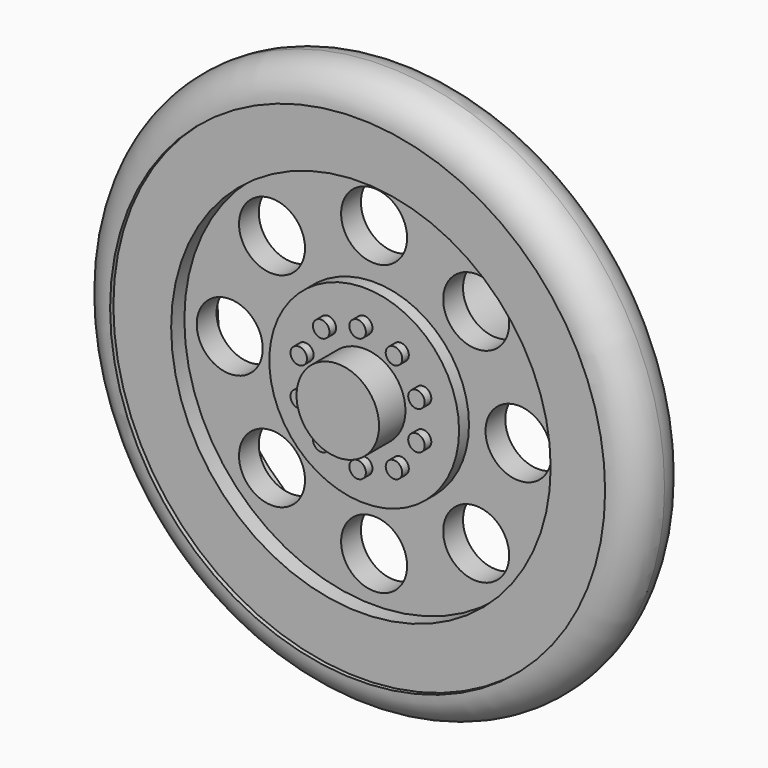
from build123d import *

# Parameters (mm, degrees)
F0_R      = 17
F1_DEPTH  = 4
F2_R      = 2
F3_R      = 1.99999
F4_R      = 15
F4_R_2    = 2
F4_R_3    = 5.75
F5_DEPTH  = 0.25
F6_DEPTH  = 0.25
F7_R      = 11.5
F7_R_2    = 2
F7_R_3    = 5.75
F8_DEPTH  = 1
F9_R      = 11.5
F10_DEPTH = 1
F11_DEPTH = 5
F12_DEPTH = 0.5
F13_R     = 0.5
F14_DEPTH = 0.5
F13_R_2   = 2.5
F15_DEPTH = 2
F16_R     = 3
F17_DEPTH = 8.5
F18_R     = 1.5
F19_DEPTH = 9


# Not quite as in the source:
# - a fillet or chamfer is up to 0.001 mm smaller than in the source, because OpenCascade refuses the exact size


with BuildPart() as f1:
    # F0 (on Front) → F1 (new body)
    with BuildSketch(Plane.XZ):
        Circle(F0_R)
    extrude(amount=F1_DEPTH)

    # F2
    f2_edges = [f1.edges().sort_by_distance(p)[0] for p in [
        (-17, -4, 0),
    ]]
    fillet(f2_edges, radius=F2_R)

    # F3 (radius 2 in the source; OpenCascade refuses exactly that, so slightly less here)
    f3_edges = [f1.edges().sort_by_distance(p)[0] for p in [
        (-17, 0, 0),
    ]]
    fillet(f3_edges, radius=F3_R)

    # F4 (on face) → F5 (cut)
    with BuildSketch(Plane.XZ.offset(4)):
        Circle(F4_R)
        with Locations((-6.1871843354, -6.1871843354)):
            Circle(F4_R_2, mode=Mode.SUBTRACT)
        with Locations((0, -8.75)):
            Circle(F4_R_2, mode=Mode.SUBTRACT)
        with Locations((6.1871843354, -6.1871843354)):
            Circle(F4_R_2, mode=Mode.SUBTRACT)
        with Locations((-8.75, 0)):
            Circle(F4_R_2, mode=Mode.SUBTRACT)
        with Locations((-6.1871843354, 6.1871843354)):
            Circle(F4_R_2, mode=Mode.SUBTRACT)
        Circle(F4_R_3, mode=Mode.SUBTRACT)
        with Locations((6.1871843354, 6.1871843354)):
            Circle(F4_R_2, mode=Mode.SUBTRACT)
        with Locations((8.75, 0)):
            Circle(F4_R_2, mode=Mode.SUBTRACT)
        with Locations((0, 8.75)):
            Circle(F4_R_2, mode=Mode.SUBTRACT)
    extrude(amount=-F5_DEPTH, mode=Mode.SUBTRACT)

    # F6 (cut): a face of the model
    f6_faces = [f1.faces().sort_by_distance(p)[0] for p in [
        (0, 0, 0),
    ]]
    extrude(f6_faces, amount=-F6_DEPTH, mode=Mode.SUBTRACT)

    # F7 (on face) → F8 (cut)
    with BuildSketch(Plane.XZ.offset(3.75)):
        Circle(F7_R)
        with Locations((-6.1871843354, -6.1871843354)):
            Circle(F7_R_2, mode=Mode.SUBTRACT)
        with Locations((0, -8.75)):
            Circle(F7_R_2, mode=Mode.SUBTRACT)
        with Locations((6.1871843354, -6.1871843354)):
            Circle(F7_R_2, mode=Mode.SUBTRACT)
        with Locations((-8.75, 0)):
            Circle(F7_R_2, mode=Mode.SUBTRACT)
        with Locations((-6.1871843354, 6.1871843354)):
            Circle(F7_R_2, mode=Mode.SUBTRACT)
        Circle(F7_R_3, mode=Mode.SUBTRACT)
        with Locations((6.1871843354, 6.1871843354)):
            Circle(F7_R_2, mode=Mode.SUBTRACT)
        with Locations((8.75, 0)):
            Circle(F7_R_2, mode=Mode.SUBTRACT)
        with Locations((0, 8.75)):
            Circle(F7_R_2, mode=Mode.SUBTRACT)
    extrude(amount=-F8_DEPTH, mode=Mode.SUBTRACT)

    # F9 (on face) → F10 (cut)
    with BuildSketch(Plane(origin=(0, -0.25, 0), x_dir=(-1, 0, 0), z_dir=(0, 1, 0))):
        Circle(F9_R)
    extrude(amount=-F10_DEPTH, mode=Mode.SUBTRACT)

    # F11 (cut): faces of the model
    f11_faces = [f1.faces().sort_by_distance(p)[0] for p in [
        (-6.1871843354, -4, 6.1871843354),
        (0, -4, 8.75),
        (6.1871843354, -4, 6.1871843354),
        (8.75, -4, 0),
        (6.1871843354, -4, -6.1871843354),
        (0, -4, -8.75),
        (-6.1871843354, -4, -6.1871843354),
        (-8.75, -4, 0),
    ]]
    extrude(f11_faces, amount=-F11_DEPTH, mode=Mode.SUBTRACT)

    # F12 (cut): a face of the model
    f12_faces = [f1.faces().sort_by_distance(p)[0] for p in [
        (0, -4, 0),
    ]]
    extrude(f12_faces, amount=-F12_DEPTH, mode=Mode.SUBTRACT)

    # F13 (on face) → F14 (join)
    with BuildSketch(Plane.XZ.offset(3.5)):
        with Locations((0, 3.75)):
            Circle(F13_R)
        with Locations((2.2041946961, 3.0338137289)):
            Circle(F13_R)
        with Locations((3.5664619361, 1.1588137289)):
            Circle(F13_R)
        with Locations((3.5664619361, -1.1588137289)):
            Circle(F13_R)
        with Locations((2.2041946961, -3.0338137289)):
            Circle(F13_R)
        with Locations((0, -3.75)):
            Circle(F13_R)
        with Locations((-2.2041946961, -3.0338137289)):
            Circle(F13_R)
        with Locations((-3.5664619361, -1.1588137289)):
            Circle(F13_R)
        with Locations((-3.5664619361, 1.1588137289)):
            Circle(F13_R)
        with Locations((-2.2041946961, 3.0338137289)):
            Circle(F13_R)
    extrude(amount=F14_DEPTH)

    # F13 (on face) → F15 (join)
    with BuildSketch(Plane.XZ.offset(3.5)):
        Circle(F13_R_2)
    extrude(amount=F15_DEPTH)

    # F16 (on face) → F17 (join)
    with BuildSketch(Plane(origin=(0, -1.25, 0), x_dir=(-1, 0, 0), z_dir=(0, 1, 0))):
        Circle(F16_R)
    extrude(amount=F17_DEPTH)

    # F18 (on face) → F19 (cut)
    with BuildSketch(Plane(origin=(0, 7.25, 0), x_dir=(-1, 0, 0), z_dir=(0, 1, 0))):
        Circle(F18_R)
    extrude(amount=-F19_DEPTH, mode=Mode.SUBTRACT)


solid = f1.part
